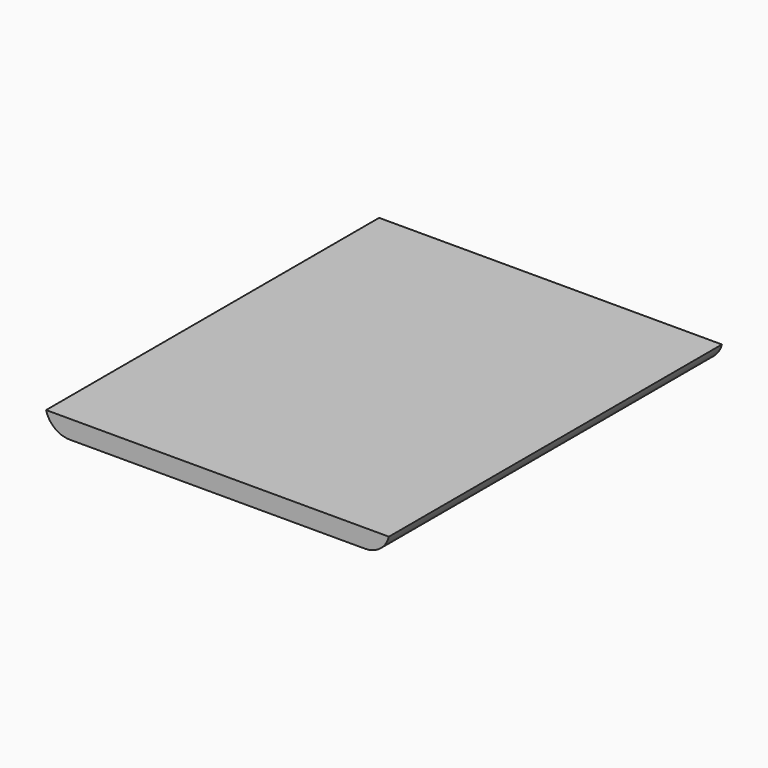
from build123d import *

# Parameters (mm, degrees)
F0_W        = 14
F0_H        = 17
F1_DEPTH    = 0.75
F2_T1_DEPTH = 21.8412291828


# Not quite as in the source:
# - a fillet or chamfer that OpenCascade refuses, or shapes differently, is made with other operations: its cross-section is extruded or revolved along the edge and cut away or added


with BuildPart() as f1:
    # F0 (on Top) → F1 (new body)
    with BuildSketch(Plane.XY):
        with Locations((7, 8.5)):
            Rectangle(F0_W, F0_H)
    extrude(amount=F1_DEPTH)

    # F2: fillet of radius 1 on 2 edges, made by hand

    # F2_s2 → F2_t1 (cut)
    with BuildSketch(Plane.XZ.offset(-19.4206145914)):
        with BuildLine():
            ThreePointArc((14, 0.75), (13.6441265991, 0.209430585), (13.0317541634, 0))
            Line((13.0317541634, 0), (14, 0))
            Line((14, 0), (14, 0.75))
        make_face()
        with BuildLine():
            ThreePointArc((0, 0.75), (0.3558734009, 0.209430585), (0.9682458366, 0))
            Line((0.9682458366, 0), (0, 0))
            Line((0, 0), (0, 0.75))
        make_face()
    extrude(amount=F2_T1_DEPTH, mode=Mode.SUBTRACT)


solid = f1.part
